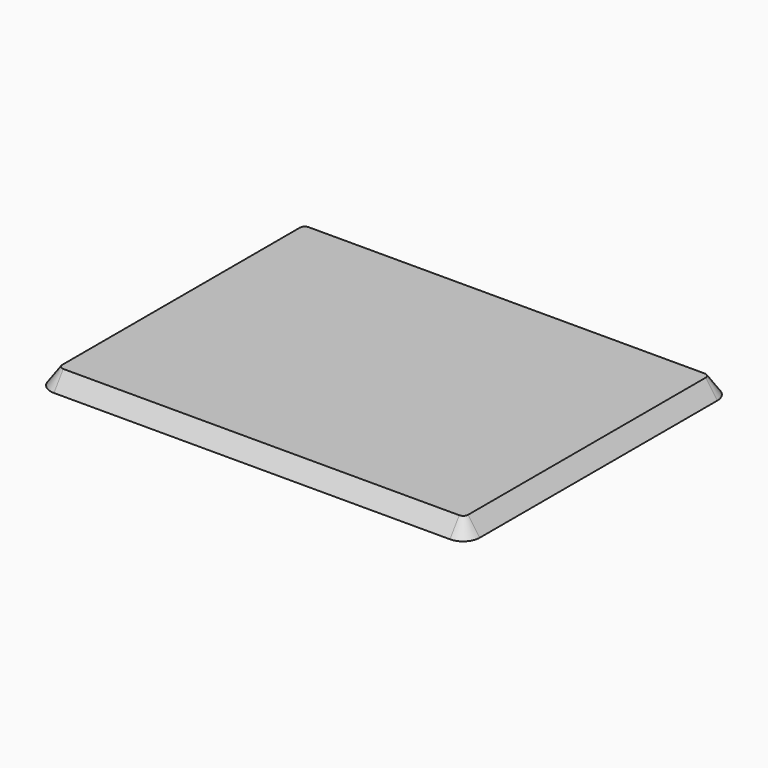
from build123d import *

# Parameters (mm, degrees)
F0_W     = 65
F0_H     = 50
F1_DEPTH = 2.5
F2_R     = 2.5
F3_SIZE2 = 2.49999
F3_SIZE  = 1.750509


# Not quite as in the source:
# - a fillet or chamfer is up to 0.001 mm smaller than in the source, because OpenCascade refuses the exact size


with BuildPart() as f1:
    # F0 (on Top) → F1 (new body)
    with BuildSketch(Plane.XY):
        Rectangle(F0_W, F0_H)
    extrude(amount=F1_DEPTH)

    # F2
    f2_edges = [f1.edges().sort_by_distance(p)[0] for p in [
        (-32.5, -25, 1.25),
        (32.5, -25, 1.25),
        (32.5, 25, 1.25),
        (-32.5, 25, 1.25),
    ]]
    fillet(f2_edges, radius=F2_R)

    # F3 (size 1.7505188455 and 2.5 in the source; OpenCascade refuses exactly that, so slightly less here)
    f3_edges = [f1.edges().sort_by_distance(p)[0] for p in [
        (-32.5, 0, 2.5),
        (-31.767767, 24.267767, 2.5),
        (0, 25, 2.5),
        (31.767767, 24.267767, 2.5),
        (32.5, 0, 2.5),
        (31.767767, -24.267767, 2.5),
        (0, -25, 2.5),
        (-31.767767, -24.267767, 2.5),
    ]]
    f3_side = f1.faces().sort_by_distance((0, 0, 2.5))[0]
    chamfer(f3_edges, length=F3_SIZE, length2=F3_SIZE2, reference=f3_side)


solid = f1.part
